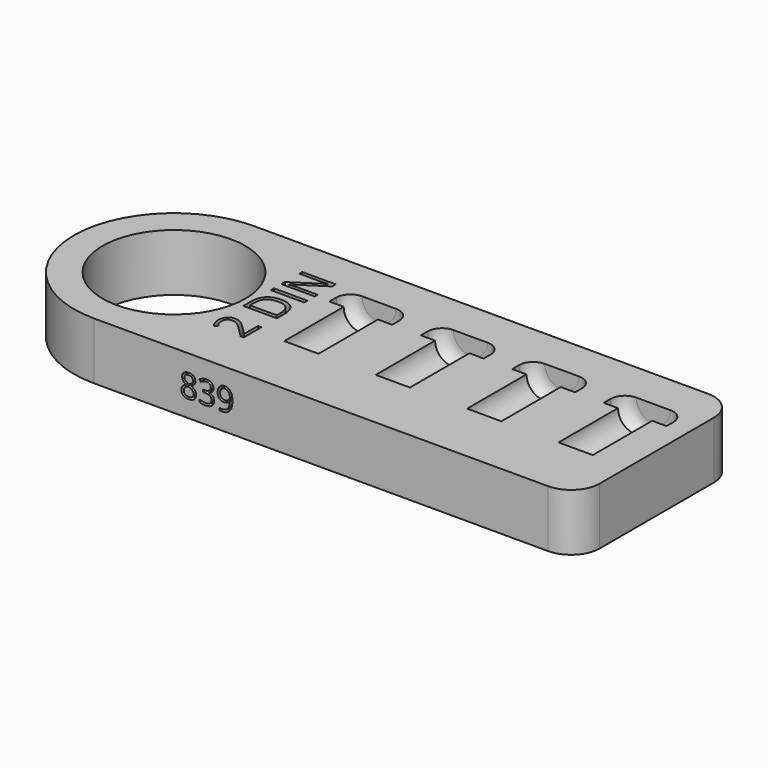
from build123d import *

# Parameters (mm, degrees)
F0_R          = 12.5
F1_DEPTH      = 10
F2_TEXT_SIZE  = 8.2204057172
F7_DEPTH      = 2
F8_TEXT_SIZE  = 8.3433869986
F9_DEPTH      = 2
F12_TEXT_SIZE = 5.5555555556
F13_DEPTH     = 1


# Not quite as in the source:
# - Text() gives the source's letters only with a copy of the font that has no kerning and outlines rounded to 1/6400 em; it was checked with that copy


with BuildPart() as f1:
    # F0 (on Top) → F1 (new body)
    with BuildSketch(Plane.XY):
        with BuildLine():
            ThreePointArc((0, 17.5), (5.1256313292, 5.1256313292), (17.5, 0))
            Line((17.5, 0), (97, 0))
            ThreePointArc((97, 0), (100.5355339059, 1.4644660941), (102, 5))
            Line((102, 5), (102, 30))
            ThreePointArc((102, 30), (100.5355339059, 33.5355339059), (97, 35))
            Line((97, 35), (17.5, 35))
            ThreePointArc((17.5, 35), (5.1256313292, 29.8743686708), (0, 17.5))
        make_face()
        with Locations((17.5, 17.5)):
            Circle(F0_R, mode=Mode.SUBTRACT)
    extrude(amount=F1_DEPTH)

    # F2 (on face) → F3 (revolve, cut)
    with BuildSketch(Plane.XY.offset(10)):
        with BuildLine():
            Line((45, 24), (45, 11))
            Line((45, 11), (48, 11))
            Line((48, 11), (48, 24))
            Line((48, 24), (50.5, 24))
            Line((50.5, 24), (50.5, 25.5))
            ThreePointArc((50.5, 25.5), (49.767766953, 27.267766953), (48, 28))
            Line((48, 28), (45, 28))
            Line((45, 28), (45, 24))
        make_face()
    revolve(axis=Axis((45, 17.5, 10), (0, 1, 0)), mode=Mode.SUBTRACT)

    # F2 (on face) → F4 (revolve, cut)
    with BuildSketch(Plane.XY.offset(10)):
        with BuildLine():
            Line((61, 24), (61, 11))
            Line((61, 11), (64, 11))
            Line((64, 11), (64, 24))
            Line((64, 24), (66.5, 24))
            Line((66.5, 24), (66.5, 25.5))
            ThreePointArc((66.5, 25.5), (65.767766953, 27.267766953), (64, 28))
            Line((64, 28), (61, 28))
            Line((61, 28), (61, 24))
        make_face()
    revolve(axis=Axis((61, 17.5, 10), (0, 1, 0)), mode=Mode.SUBTRACT)

    # F2 (on face) → F5 (revolve, cut)
    with BuildSketch(Plane.XY.offset(10)):
        with BuildLine():
            Line((77, 24), (77, 11))
            Line((77, 11), (80, 11))
            Line((80, 11), (80, 24))
            Line((80, 24), (82.5, 24))
            Line((82.5, 24), (82.5, 25.5))
            ThreePointArc((82.5, 25.5), (81.767766953, 27.267766953), (80, 28))
            Line((80, 28), (77, 28))
            Line((77, 28), (77, 24))
        make_face()
    revolve(axis=Axis((77, 17.5, 10), (0, 1, 0)), mode=Mode.SUBTRACT)

    # F2 (on face) → F6 (revolve, cut)
    with BuildSketch(Plane.XY.offset(10)):
        with BuildLine():
            Line((93, 24), (93, 11))
            Line((93, 11), (96, 11))
            Line((96, 11), (96, 24))
            Line((96, 24), (98.5, 24))
            Line((98.5, 24), (98.5, 25.5))
            ThreePointArc((98.5, 25.5), (97.767766953, 27.267766953), (96, 28))
            Line((96, 28), (93, 28))
            Line((93, 28), (93, 24))
        make_face()
    revolve(axis=Axis((93, 17.5, 10), (0, 1, 0)), mode=Mode.SUBTRACT)

    # F2 (on face) → F7 (cut)
    with BuildSketch(Plane.XY.offset(10)):
        with Locations(Location((37, 8), (0, 0, 90))):
            Text('2 DIN', F2_TEXT_SIZE, font='Open Sans', text_align=(TextAlign.LEFT, TextAlign.BOTTOM))
    extrude(amount=-F7_DEPTH, mode=Mode.SUBTRACT)

    # F8 (on face) → F9 (cut)
    with BuildSketch(Plane(origin=(0, 0, 0), x_dir=(1, 0, 0), z_dir=(0, 0, -1))):
        with Locations(Location((37, -27), (0, 0, 90))):
            Text('1 DIN', F8_TEXT_SIZE, font='Open Sans', font_style=FontStyle.BOLD, text_align=(TextAlign.LEFT, TextAlign.BOTTOM))
    extrude(amount=-F9_DEPTH, mode=Mode.SUBTRACT)

    # F8 (on face) → F10 (revolve, cut)
    with BuildSketch(Plane(origin=(0, 0, 0), x_dir=(1, 0, 0), z_dir=(0, 0, -1))):
        with BuildLine():
            Line((47, -11), (47, -24))
            Line((47, -24), (50, -24))
            Line((50, -24), (50, -11))
            Line((50, -11), (52.5, -11))
            Line((52.5, -11), (52.5, -9.5))
            ThreePointArc((52.5, -9.5), (51.767766953, -7.732233047), (50, -7))
            Line((50, -7), (47, -7))
            Line((47, -7), (47, -11))
        make_face()
    revolve(axis=Axis((47, 17.5, 0), (0, -1, 0)), mode=Mode.SUBTRACT)

    # F8 (on face) → F11 (revolve, cut)
    with BuildSketch(Plane(origin=(0, 0, 0), x_dir=(1, 0, 0), z_dir=(0, 0, -1))):
        with BuildLine():
            Line((63, -11), (63, -24))
            Line((63, -24), (66, -24))
            Line((66, -24), (66, -11))
            Line((66, -11), (68.5, -11))
            Line((68.5, -11), (68.5, -9.5))
            ThreePointArc((68.5, -9.5), (67.767766953, -7.732233047), (66, -7))
            Line((66, -7), (63, -7))
            Line((63, -7), (63, -11))
        make_face()
    revolve(axis=Axis((63, 17.5, 0), (0, -1, 0)), mode=Mode.SUBTRACT)

    # F12 (on face) → F13 (cut)
    with BuildSketch(Plane.XZ):
        with Locations((32.5, 3)):
            Text('839', F12_TEXT_SIZE, font='Open Sans', text_align=(TextAlign.LEFT, TextAlign.BOTTOM))
    extrude(amount=-F13_DEPTH, mode=Mode.SUBTRACT)


solid = f1.part
